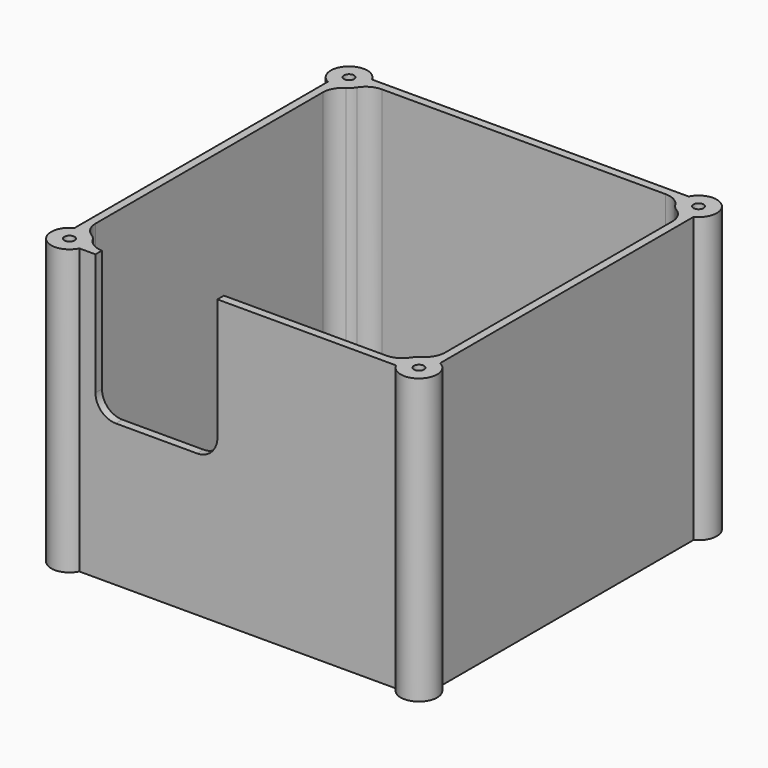
from build123d import *

# Parameters (mm, degrees)
F0_W          = 90
F0_H          = 90
F1_DEPTH      = 70
F2_W          = 86
F2_H          = 86
F3_DEPTH      = 65
F4_R          = 4.5
F5_DEPTH      = 70
F6_W          = 30
F6_H          = 35
F7_DEPTH      = 2
F8_R          = 1.25
F9_DEPTH      = 15
F10_R         = 4
F10_R_2       = 1.25
F11_DEPTH     = 13
F12_T1_DEPTH  = 2
F12_T3_DEPTH  = 65
F12_T8_DEPTH  = 73.9443680268
F12_T13_DEPTH = 65


# Not quite as in the source:
# - a fillet or chamfer that OpenCascade refuses, or shapes differently, is made with other operations: its cross-section is extruded or revolved along the edge and cut away or added
# - a feature of the source that left no trace in its solid (it failed there, or was rolled back) is left out


with BuildPart() as f1:
    # F0 (on Top) → F1 (new body)
    with BuildSketch(Plane.XY):
        with Locations((45, 45)):
            Rectangle(F0_W, F0_H)
    extrude(amount=F1_DEPTH)

    # F2 (on face) → F3 (cut)
    with BuildSketch(Plane.XY.offset(70)):
        with Locations((45, 45)):
            Rectangle(F2_W, F2_H)
    extrude(amount=-F3_DEPTH, mode=Mode.SUBTRACT)

    # F4 (on Top) → F5 (join)
    with BuildSketch(Plane.XY):
        with Locations((2, 88)):
            Circle(F4_R)
        with Locations((88, 88)):
            Circle(F4_R)
        with Locations((2, 2)):
            Circle(F4_R)
        with Locations((88, 2)):
            Circle(F4_R)
    extrude(amount=F5_DEPTH)

    # F6 (on Front) → F7 (cut, through all)
    with BuildSketch(Plane.XZ):
        with Locations((25, 52.5)):
            Rectangle(F6_W, F6_H)
    extrude(amount=-F7_DEPTH, mode=Mode.SUBTRACT)

    # F8 (on face) → F9 (cut)
    with BuildSketch(Plane.XY.offset(70)):
        with Locations((2, 88)):
            Circle(F8_R)
        with Locations((88, 88)):
            Circle(F8_R)
        with Locations((2, 2)):
            Circle(F8_R)
        with Locations((88, 2)):
            Circle(F8_R)
    extrude(amount=-F9_DEPTH, mode=Mode.SUBTRACT)

    # F10 (on face) → F11 (join)
    with BuildSketch(Plane.XY.offset(5)):
        with Locations((19, 73)):
            Circle(F10_R)
        with Locations((19, 73)):
            Circle(F10_R_2, mode=Mode.SUBTRACT)
        with Locations((83, 73)):
            Circle(F10_R)
        with Locations((83, 73)):
            Circle(F10_R_2, mode=Mode.SUBTRACT)
        with Locations((83, 14)):
            Circle(F10_R)
        with Locations((83, 14)):
            Circle(F10_R_2, mode=Mode.SUBTRACT)
        with Locations((19, 14)):
            Circle(F10_R)
        with Locations((19, 14)):
            Circle(F10_R_2, mode=Mode.SUBTRACT)
    extrude(amount=F11_DEPTH)

    # F12: fillet of radius 5 on 10 edges, made by hand

    # F12_s2 → F12_t1 (join)
    with BuildSketch(Plane.XZ.offset(-2)):
        with BuildLine():
            ThreePointArc((40, 40), (38.5355339059, 36.4644660941), (35, 35))
            Line((35, 35), (40, 35))
            Line((40, 35), (40, 40))
        make_face()
        with BuildLine():
            ThreePointArc((15, 35), (11.4644660941, 36.4644660941), (10, 40))
            Line((10, 40), (10, 35))
            Line((10, 35), (15, 35))
        make_face()
    extrude(amount=F12_T1_DEPTH)

    # F12_s4 → F12_t3 (join)
    with BuildSketch(Plane.XY.offset(5)):
        with BuildLine():
            ThreePointArc((79.9222527893, 2), (82.3555741063, 2.6320545598), (84.1736986897, 4.3684210526))
            ThreePointArc((84.1736986897, 4.3684210526), (83.6717003398, 3.2311872529), (83.5, 2))
            Line((83.5, 2), (79.9222527893, 2))
        make_face()
        with BuildLine():
            ThreePointArc((85.6315789474, 5.8263013103), (87.3679454402, 7.6444258937), (88, 10.0777472107))
            Line((88, 10.0777472107), (88, 6.5))
            ThreePointArc((88, 6.5), (86.7688127471, 6.3282996602), (85.6315789474, 5.8263013103))
        make_face()
        with BuildLine():
            ThreePointArc((4.3684210526, 5.8263013103), (2.6320545598, 7.6444258937), (2, 10.0777472107))
            Line((2, 10.0777472107), (2, 6.5))
            ThreePointArc((2, 6.5), (3.2311872529, 6.3282996602), (4.3684210526, 5.8263013103))
        make_face()
        with BuildLine():
            ThreePointArc((88, 79.9222527893), (87.3679454402, 82.3555741063), (85.6315789474, 84.1736986897))
            ThreePointArc((85.6315789474, 84.1736986897), (86.7688127471, 83.6717003398), (88, 83.5))
            Line((88, 83.5), (88, 79.9222527893))
        make_face()
        with BuildLine():
            ThreePointArc((2, 79.9222527893), (2.6320545598, 82.3555741063), (4.3684210526, 84.1736986897))
            ThreePointArc((4.3684210526, 84.1736986897), (3.2311872529, 83.6717003398), (2, 83.5))
            Line((2, 83.5), (2, 79.9222527893))
        make_face()
        with BuildLine():
            ThreePointArc((84.1736986897, 85.6315789474), (82.3555741063, 87.3679454402), (79.9222527893, 88))
            Line((79.9222527893, 88), (83.5, 88))
            ThreePointArc((83.5, 88), (83.6717003398, 86.7688127471), (84.1736986897, 85.6315789474))
        make_face()
        with BuildLine():
            ThreePointArc((5.8263013103, 85.6315789474), (7.6444258937, 87.3679454402), (10.0777472107, 88))
            Line((10.0777472107, 88), (6.5, 88))
            ThreePointArc((6.5, 88), (6.3282996602, 86.7688127471), (5.8263013103, 85.6315789474))
        make_face()
    extrude(amount=F12_T3_DEPTH)


with BuildPart() as f12_tool6:
    # F12_s7 → F12_t8 (new body)
    with BuildSketch(Plane.XY.offset(5)):
        with BuildLine():
            ThreePointArc((10.0777472107, 2), (7.6444258937, 2.6320545598), (5.8263013103, 4.3684210526))
            ThreePointArc((5.8263013103, 4.3684210526), (6.3282996602, 3.2311872529), (6.5, 2))
            Line((6.5, 2), (10.0777472107, 2))
        make_face()
    extrude(amount=F12_T8_DEPTH)

    split(bisect_by=Plane.XY.offset(35), keep=Keep.BOTTOM)


with BuildPart() as f1_1:
    add(f1.part)

    # F12_t5: union F12_tool6
    add(f12_tool6.part)


with BuildPart() as f12_tool11:
    # F12_s12 → F12_t13 (new body)
    with BuildSketch(Plane.XY.offset(5)):
        with BuildLine():
            ThreePointArc((10.0777472107, 2), (7.6444258937, 2.6320545598), (5.8263013103, 4.3684210526))
            ThreePointArc((5.8263013103, 4.3684210526), (6.3282996602, 3.2311872529), (6.5, 2))
            Line((6.5, 2), (10.0777472107, 2))
        make_face()
    extrude(amount=F12_T13_DEPTH)

    split(bisect_by=Plane.YZ.offset(10), keep=Keep.BOTTOM)


with BuildPart() as f1_2:
    add(f1_1.part)

    # F12_t10: union F12_tool11
    add(f12_tool11.part)


solid = f1_2.part
